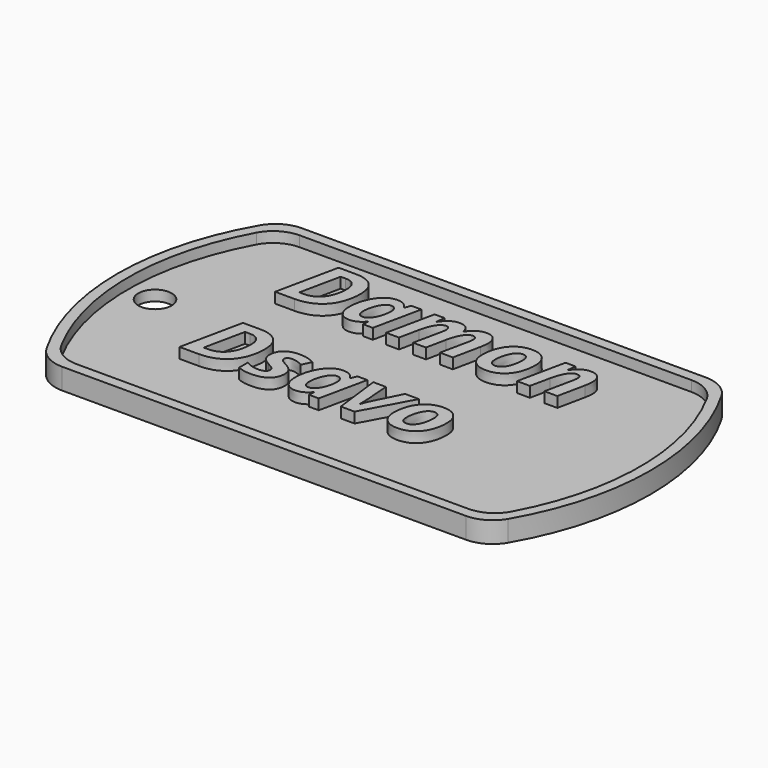
from build123d import *

# Parameters (mm, degrees)
F1_DEPTH     = 1
F3_DEPTH     = 1
F4_R         = 1.5875
F5_DEPTH     = 1
F6_TEXT_SIZE = 8.3729065308
F7_DEPTH     = 1


# Not quite as in the source:
# - Text() gives the source's letters only with a copy of the font that has no kerning and outlines rounded to 1/6400 em; it was checked with that copy


with BuildPart() as f1:
    # F0 (on Top) → F1 (new body)
    with BuildSketch(Plane.XY):
        with BuildLine():
            ThreePointArc((-19.2474145991, 14.2875), (-20.8349145991, 13.862130657), (-21.9970452561, 12.7))
            ThreePointArc((-21.9970452561, 12.7), (-25.4, 0), (-21.9970452561, -12.7))
            ThreePointArc((-21.9970452561, -12.7), (-20.8349145991, -13.862130657), (-19.2474145991, -14.2875))
            Line((-19.2474145991, -14.2875), (19.2474145991, -14.2875))
            ThreePointArc((19.2474145991, -14.2875), (20.8349145991, -13.862130657), (21.9970452561, -12.7))
            ThreePointArc((21.9970452561, -12.7), (25.4, 0), (21.9970452561, 12.7))
            ThreePointArc((21.9970452561, 12.7), (20.8349145991, 13.862130657), (19.2474145991, 14.2875))
            Line((19.2474145991, 14.2875), (-19.2474145991, 14.2875))
        make_face()
    extrude(amount=F1_DEPTH)

    # F2 (on face) → F3 (join)
    with BuildSketch(Plane.XY.offset(1)):
        with BuildLine():
            Line((19.2474145991, 14.2875), (-19.2474145991, 14.2875))
            ThreePointArc((-19.2474145991, 14.2875), (-20.8349145991, 13.862130657), (-21.9970452561, 12.7))
            ThreePointArc((-21.9970452561, 12.7), (-25.4, 0), (-21.9970452561, -12.7))
            ThreePointArc((-21.9970452561, -12.7), (-20.8349145991, -13.862130657), (-19.2474145991, -14.2875))
            Line((-19.2474145991, -14.2875), (19.2474145991, -14.2875))
            ThreePointArc((19.2474145991, -14.2875), (20.8349145991, -13.862130657), (21.9970452561, -12.7))
            ThreePointArc((21.9970452561, -12.7), (25.4, 0), (21.9970452561, 12.7))
            ThreePointArc((21.9970452561, 12.7), (20.8349145991, 13.862130657), (19.2474145991, 14.2875))
        make_face()
        with BuildLine():
            ThreePointArc((-21.4526124879, 11.6252061249), (-20.2856017842, 12.8404540819), (-18.6611352482, 13.2875))
            Line((-18.6611352482, 13.2875), (18.6611352482, 13.2875))
            ThreePointArc((18.6611352482, 13.2875), (20.2856017842, 12.8404540819), (21.4526124879, 11.6252061249))
            ThreePointArc((21.4526124879, 11.6252061249), (24.4, 0), (21.4526124879, -11.6252061249))
            ThreePointArc((21.4526124879, -11.6252061249), (20.2856017842, -12.8404540819), (18.6611352482, -13.2875))
            Line((18.6611352482, -13.2875), (-18.6611352482, -13.2875))
            ThreePointArc((-18.6611352482, -13.2875), (-20.2856017842, -12.8404540819), (-21.4526124879, -11.6252061249))
            ThreePointArc((-21.4526124879, -11.6252061249), (-24.4, 0), (-21.4526124879, 11.6252061249))
        make_face(mode=Mode.SUBTRACT)
    extrude(amount=F3_DEPTH)

    # F4 (on face) → F5 (cut)
    with BuildSketch(Plane.XY.offset(1)):
        with Locations((-21.821282804, 0)):
            Circle(F4_R)
    extrude(amount=-F5_DEPTH, mode=Mode.SUBTRACT)


with BuildPart() as f7:
    # F6 (on face) → F7 (new body)
    with BuildSketch(Plane.XY.offset(2)):
        with Locations((-13.4306550026, 3.5445189569)):
            Text('Damon', F6_TEXT_SIZE, font='Open Sans', font_style=FontStyle.BOLDITALIC, text_align=(TextAlign.LEFT, TextAlign.BOTTOM))
        with Locations((-13.4306550026, -7.842633925)):
            Text('Dsavo', F6_TEXT_SIZE, font='Open Sans', font_style=FontStyle.BOLDITALIC, text_align=(TextAlign.LEFT, TextAlign.BOTTOM))
    extrude(amount=F7_DEPTH)


solid = Compound([f1.part, f7.part])
